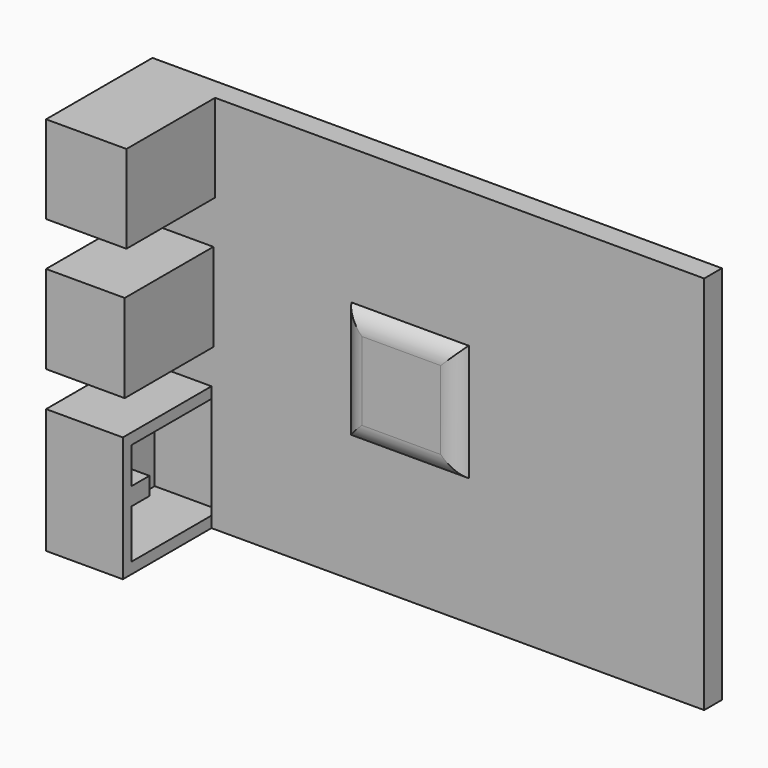
from build123d import *

# Parameters (mm, degrees)
F0_W         = 130.5194124579
F0_H         = 87.0954208076
F1_DEPTH     = 5.08
F2_W         = 18.4217169881
F2_H         = 20.1326627284
F3_DEPTH     = 25.4
F4_W         = 18.0227532983
F4_H         = 20.2161408961
F5_DEPTH     = 25.4
F6_W         = 17.5940208137
F6_H         = 28.6207161844
F7_DEPTH     = 25.4
F8_T         = 2.54
F8_T3_DEPTH  = 22.6740208137
F8_T5_DEPTH  = 23.1027532983
F8_T7_DEPTH  = 25.2961408961
F8_T9_DEPTH  = 23.5017169881
F8_T11_DEPTH = 25.2126627284
F9_W         = 15.0540208137
F9_H         = 4.0768496692
F10_DEPTH    = 5.08
F11_W        = 26.8854014575
F11_H        = 26.7390697263
F12_DEPTH    = 2.54
F13_T1_DEPTH = 48.8824467137
F13_T3_DEPTH = 48.7361149824


# Not quite as in the source:
# - a fillet or chamfer that OpenCascade refuses, or shapes differently, is made with other operations: its cross-section is extruded or revolved along the edge and cut away or added
# - a shell that OpenCascade refuses in one call is made with other operations: the cavity is built on its own and cut out


with BuildPart() as f1:
    # F0 (on Front) → F1 (new body)
    with BuildSketch(Plane.XZ):
        with Locations((2.1416731179, -2.8366688639)):
            Rectangle(F0_W, F0_H)
    extrude(amount=F1_DEPTH)

    # F2 (on face) → F3 (join)
    with BuildSketch(Plane.XZ.offset(5.08)):
        with Locations((-53.9071746171, 30.6447101757)):
            Rectangle(F2_W, F2_H)
    extrude(amount=F3_DEPTH)

    # F4 (on face) → F5 (join)
    with BuildSketch(Plane.XZ.offset(5.08)):
        with Locations((-54.106656462, 0.4099132493)):
            Rectangle(F4_W, F4_H)
    extrude(amount=F5_DEPTH)

    # F6 (on face) → F7 (join)
    with BuildSketch(Plane.XZ.offset(5.08)):
        with Locations((-54.3210227042, -32.0740211755)):
            Rectangle(F6_W, F6_H)
    extrude(amount=F7_DEPTH)

    # F8: shell of thickness 2.54, made by hand


with BuildPart() as f8_core1:
    # F8_t2: copy of F1
    add(f1.part)

    # the walls: a layer under each face that stays
    f8_faces = [f8_core1.faces().sort_by_distance(p)[0] for p in [
        (-63.1180331111, -15.24, -2.8366688639),
        (2.1416731179, 0, -2.8366688639),
        (67.4013793468, -2.54, -2.8366688639),
        (-53.7952179355, -28.3028571429, -46.3843792677),
        (-54.3210227042, -30.48, -32.0740211755),
        (-54.3210227042, -17.78, -17.7636630833),
        (-54.106656462, -17.78, -9.6981571987),
        (-45.0952798128, -17.78, 0.4099132493),
        (-54.106656462, -30.48, 0.4099132493),
        (-54.106656462, -17.78, 10.5179836974),
        (2.1416731179, -5.08, -2.8366688639),
        (-44.696316123, -17.78, 30.6447101757),
        (-53.9071746171, -17.78, 20.5783788115),
        (-53.9071746171, -30.48, 30.6447101757),
        (58.0785641713, -2.1771428571, 40.7110415399),
    ]]
    thicken(f8_faces, amount=-F8_T, mode=Mode.SUBTRACT)

    # F8_s4 → F8_t3 (cut)
    with BuildSketch(Plane.YZ.offset(-65.6580331111)):
        Polygon((-5.1054, -17.7382630833), (-5.08, -20.3036630833), (-2.54, -20.3036630833), (-2.54, -17.7636630833), align=None)
    extrude(amount=F8_T3_DEPTH, mode=Mode.SUBTRACT)

    # F8_s6 → F8_t5 (cut)
    with BuildSketch(Plane.YZ.offset(-65.6580331111)):
        Polygon((-5.1054, -9.7235571987), (-5.08, -7.1581571987), (-2.54, -7.1581571987), (-2.54, -9.6981571987), align=None)
        Polygon((-5.1054, 10.5433836974), (-5.08, 7.9779836974), (-2.54, 7.9779836974), (-2.54, 10.5179836974), align=None)
    extrude(amount=F8_T5_DEPTH, mode=Mode.SUBTRACT)

    # F8_s8 → F8_t7 (cut)
    with BuildSketch(Plane.XY.offset(-12.2381571987)):
        Polygon((-45.0698798128, -5.1054), (-47.6352798128, -5.08), (-47.6352798128, -2.54), (-45.0952798128, -2.54), align=None)
    extrude(amount=F8_T7_DEPTH, mode=Mode.SUBTRACT)

    # F8_s10 → F8_t9 (cut)
    with BuildSketch(Plane.YZ.offset(-65.6580331111)):
        Polygon((-5.1054, 20.5529788115), (-2.54, 20.5783788115), (-2.54, 23.1183788115), (-5.08, 23.1183788115), align=None)
    extrude(amount=F8_T9_DEPTH, mode=Mode.SUBTRACT)

    # F8_s12 → F8_t11 (cut)
    with BuildSketch(Plane.XY.offset(18.0383788115)):
        Polygon((-44.670916123, -5.1054), (-44.696316123, -2.54), (-47.236316123, -2.54), (-47.236316123, -5.08), align=None)
    extrude(amount=F8_T11_DEPTH, mode=Mode.SUBTRACT)


with BuildPart() as f1_1:
    add(f1.part)

    # what is left inside the walls is the cavity
    f8_cavity = [f8_core1.part.solids().sort_by_distance(p)[0] for p in [
        (-60.552633, -19.473333, 30.64471),
        (-60.552633, -19.473333, -32.074021),
        (-60.552633, -19.473333, 0.409913),
    ]]
    add(f8_cavity, mode=Mode.SUBTRACT)

    # F9 (on face) → F10 (join)
    with BuildSketch(Plane(origin=(0, -27.94, 0), x_dir=(-1, 0, 0), z_dir=(0, 1, 0))):
        with Locations((53.0510227042, -30.6365806609)):
            Rectangle(F9_W, F9_H)
    extrude(amount=F10_DEPTH)

    # F11 (on face) → F12 (join)
    with BuildSketch(Plane.XZ.offset(5.08)):
        with Locations((0, -3.7744471338)):
            Rectangle(F11_W, F11_H)
    extrude(amount=F12_DEPTH)

    # F13: fillet of radius 5.08 on 4 edges, made by hand

    # F13_s2 → F13_t1 (cut)
    with BuildSketch(Plane.YZ.offset(-24.4412233568)):
        with BuildLine():
            ThreePointArc((-5.08, -17.1439819969), (-6.9394090512, -15.2845729457), (-7.62, -12.7445729457))
            Line((-7.62, -12.7445729457), (-7.62, -17.1439819969))
            Line((-7.62, -17.1439819969), (-5.08, -17.1439819969))
        make_face()
        with BuildLine():
            ThreePointArc((-5.08, 9.5950877294), (-6.9394090512, 7.7356786782), (-7.62, 5.1956786782))
            Line((-7.62, 5.1956786782), (-7.62, 9.5950877294))
            Line((-7.62, 9.5950877294), (-5.08, 9.5950877294))
        make_face()
    extrude(amount=F13_T1_DEPTH, mode=Mode.SUBTRACT)

    # F13_s4 → F13_t3 (cut)
    with BuildSketch(Plane.XY.offset(-28.142504625)):
        with BuildLine():
            ThreePointArc((-13.4427007288, -5.08), (-11.5832916775, -6.9394090512), (-9.0432916775, -7.62))
            Line((-9.0432916775, -7.62), (-13.4427007288, -7.62))
            Line((-13.4427007288, -7.62), (-13.4427007288, -5.08))
        make_face()
        with BuildLine():
            ThreePointArc((13.4427007288, -5.08), (11.5832916775, -6.9394090512), (9.0432916775, -7.62))
            Line((9.0432916775, -7.62), (13.4427007288, -7.62))
            Line((13.4427007288, -7.62), (13.4427007288, -5.08))
        make_face()
    extrude(amount=F13_T3_DEPTH, mode=Mode.SUBTRACT)


solid = f1_1.part
